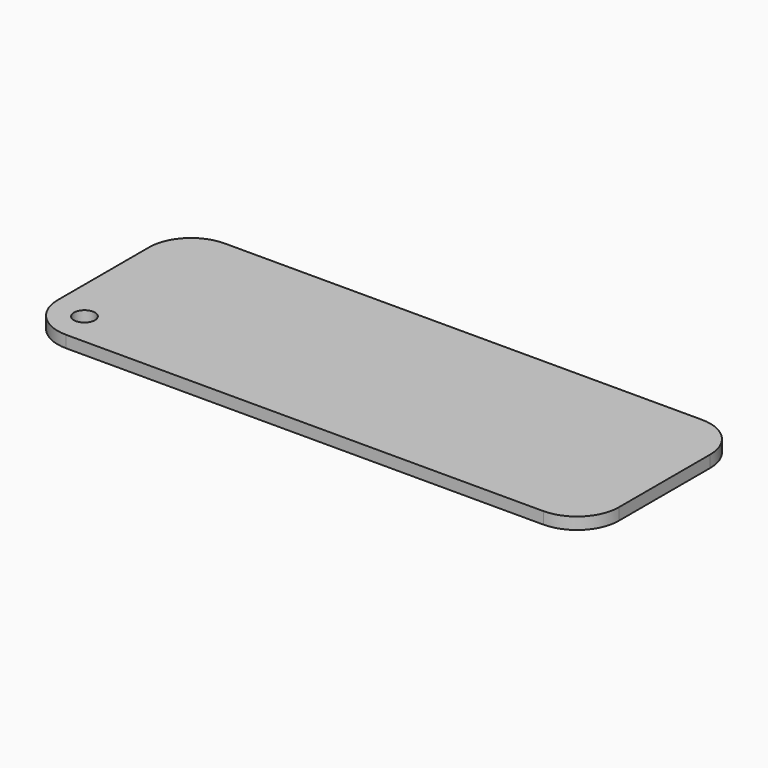
from build123d import *

# Parameters (mm, degrees)
F1_DEPTH     = 1.8
F2_R         = 1.5875
F3_DEPTH     = 25.4
F4_TEXT_SIZE = 6.6445943184
F5_DEPTH     = 1


# Not quite as in the source:
# - Text() gives the source's letters only with a copy of the font that has no kerning and outlines rounded to 1/6400 em; it was checked with that copy


with BuildPart() as f1:
    # F0 (on Top) → F1 (new body)
    with BuildSketch(Plane.XY):
        with BuildLine():
            Line((39.5632227302, 15.9403302557), (-32.7367772698, 15.9403302557))
            ThreePointArc((-32.7367772698, 15.9403302557), (-37.2269053304, 14.0804583163), (-39.0867772698, 9.5903302557))
            Line((-39.0867772698, 9.5903302557), (-39.0867772698, -7.7096697443))
            ThreePointArc((-39.0867772698, -7.7096697443), (-37.2269053304, -12.1997978048), (-32.7367772698, -14.0596697443))
            Line((-32.7367772698, -14.0596697443), (39.5632227302, -14.0596697443))
            ThreePointArc((39.5632227302, -14.0596697443), (44.0533507907, -12.1997978048), (45.9132227302, -7.7096697443))
            Line((45.9132227302, -7.7096697443), (45.9132227302, 9.5903302557))
            ThreePointArc((45.9132227302, 9.5903302557), (44.0533507907, 14.0804583163), (39.5632227302, 15.9403302557))
        make_face()
    extrude(amount=F1_DEPTH)

    # F2 (on face) → F3 (cut)
    with BuildSketch(Plane(origin=(0, 0, 0), x_dir=(1, 0, 0), z_dir=(0, 0, -1))):
        with Locations((-33.9998267591, 9.0153124183)):
            Circle(F2_R)
    extrude(amount=-F3_DEPTH, mode=Mode.SUBTRACT)

    # F4 (on face) → F5 (cut)
    with BuildSketch(Plane(origin=(0, 0, 0), x_dir=(1, 0, 0), z_dir=(0, 0, -1))):
        with Locations((-37.1965503077, -3.0100227586)):
            Text('#hackthestacks @AMNH', F4_TEXT_SIZE, font='Open Sans', font_style=FontStyle.BOLD, text_align=(TextAlign.LEFT, TextAlign.BOTTOM))
    extrude(amount=-F5_DEPTH, mode=Mode.SUBTRACT)


solid = f1.part
